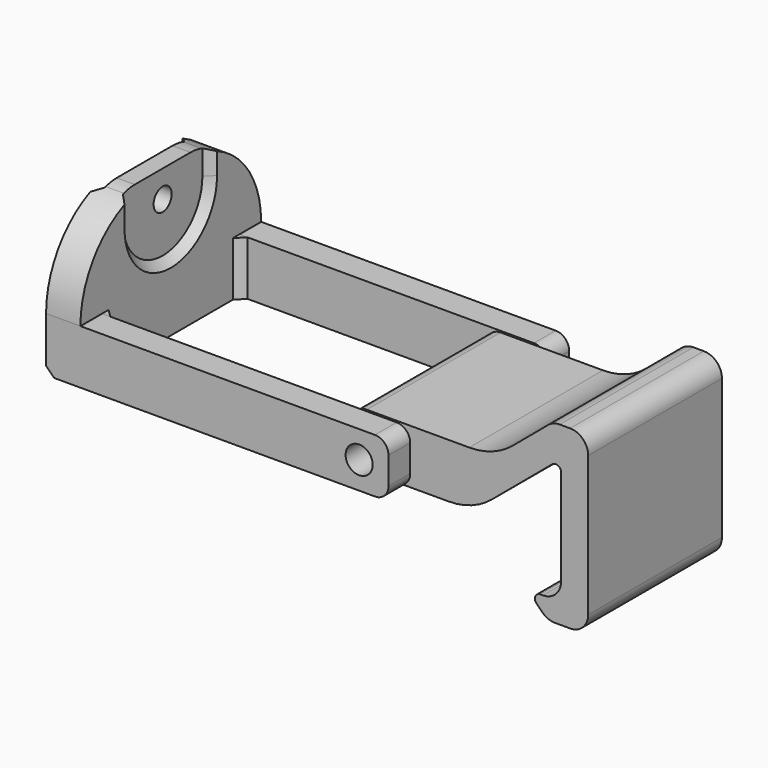
from build123d import *

# Parameters (mm, degrees)
F2_R          = 1.5
F5_DEPTH      = 12.5
F3_W          = 57.0000079349
F3_H          = 35
F3_W_2        = 5.9000002086
F3_H_2        = 3.0000003055
F6_DEPTH      = 25
F0_W          = 40
F0_H          = 30
F0_R          = 1.2500888111
F7_DEPTH      = 2
F8_DEPTH      = 1
F9_DEPTH      = 0.1
F10_DEPTH     = 0.1
F11_T4_DEPTH  = 8.3145145654
F11_T9_DEPTH  = 8.3145145654
F11_T11_DEPTH = 29.6290293933
F11_T16_ANGLE = 180
F11_T21_ANGLE = 180
F11_T26_DEPTH = 5.2499087538
F11_T31_DEPTH = 5.2499087441
F11_T36_DEPTH = 5.2499087441
F11_T41_DEPTH = 5.2499087538
F4_R          = 1.5
F12_DEPTH     = 9.25
F13_R         = 2
F14_R         = 7.5
F15_R         = 0.6
F1_W          = 40
F1_H          = 30
F16_DEPTH     = 12.5
F17_R         = 5


# Not quite as in the source:
# - a fillet or chamfer that OpenCascade refuses, or shapes differently, is made with other operations: its cross-section is extruded or revolved along the edge and cut away or added
# - ends of sketch curves that miss each other by under 0.0002 mm in the source are joined


with BuildPart() as f5:
    # F2 (on Front) → F5 (new body, symmetric)
    with BuildSketch(Plane.XZ):
        with BuildLine():
            Line((-6.5000004037, -1.225e-07), (34.4999995679, -1.225e-07))
            ThreePointArc((34.4999995679, -1.225e-07), (35.5606597229, 0.4393396988), (35.9999995441, 1.4999998538))
            Line((35.9999995441, 1.4999998538), (35.9999995441, 4.4999998063))
            ThreePointArc((35.9999995441, 4.4999998063), (35.5606597229, 5.5606599613), (34.4999995679, 5.9999997825))
            Line((34.4999995706, 5.9999997825), (1.9999998119, 5.9999998409))
            Line((1.9999998119, 5.999999905), (1.9999998119, 16))
            Line((1.9999998119, 16), (-2.000000095, 16))
            Line((-2.000000095, 16), (-2.000000095, 5.9999998557))
            Line((-2.000000095, 5.9999997745), (-6.500000401, 5.9999997825))
            ThreePointArc((-6.5000004037, 5.9999997825), (-7.5606605587, 5.5606599613), (-8.00000038, 4.4999998063))
            Line((-8.00000038, 4.4999998063), (-8.00000038, 1.4999998538))
            ThreePointArc((-8.00000038, 1.4999998538), (-7.5606605587, 0.4393396988), (-6.5000004037, -1.225e-07))
        make_face()
        with Locations((-4.7500003907, 2.9999998668)):
            Circle(F2_R, mode=Mode.SUBTRACT)
        with Locations((32.7499995548, 2.99999983)):
            Circle(F2_R, mode=Mode.SUBTRACT)
    extrude(amount=F5_DEPTH, both=True)

    # F3 (on Top) → F6 (cut)
    with BuildSketch(Plane.XY):
        with Locations((15.4999917634, -7.45e-08)):
            Rectangle(F3_W, F3_H)
        Polygon((-7.9000002086, 12.5), (-2, 12.5), (1.9999999069, 12.5), (35.9999998473, 12.5), (35.9999998473, 9.4999996945), (1.9999999069, 9.4999996945), (1.9999999069, -9.4999996945), (35.9999998473, -9.4999996945), (35.9999998473, -12.5), (1.9999999069, -12.5), (-2, -12.5), (-7.9000002086, -12.5), (-7.9000002086, -9.4999996945), (-2, -9.4999996945), (-2, 9.4999996945), (-7.9000002086, 9.4999996945), align=None, mode=Mode.SUBTRACT)
        with Locations((-4.9500001043, 10.9999998473)):
            Rectangle(F3_W_2, F3_H_2)
        with Locations((-4.9500001043, -10.9999998473)):
            Rectangle(F3_W_2, F3_H_2)
    extrude(amount=F6_DEPTH, mode=Mode.SUBTRACT)

    # F0 (on Right) → F7 (cut, symmetric)
    with BuildSketch(Plane.YZ):
        with Locations((4.47e-07, 7.9853728972)):
            Rectangle(F0_W, F0_H)
        with BuildLine():
            Line((12.5, -0.0146211902), (-12.5, -0.0146211902))
            Line((-12.5, -0.0146211902), (-12.5, 7.9853788098))
            ThreePointArc((-12.5, 7.9853788098), (-10.5000000081, 13.276881496), (-5.5, 15.9226329138))
            ThreePointArc((-5.5, 15.9226329138), (-5.000983204, 15.9696770716), (-4.4999998063, 15.9853790035))
            Line((-4.4999998063, 15.9853790035), (4.4999998063, 15.9853790035))
            ThreePointArc((4.4999998063, 15.9853790035), (5.000983204, 15.9696770716), (5.5, 15.9226329138))
            ThreePointArc((5.5, 15.9226329138), (10.5000000081, 13.276881496), (12.5, 7.9853788098))
            Line((12.5, 7.9853788098), (12.5, -0.0146211902))
        make_face(mode=Mode.SUBTRACT)
        with BuildLine():
            ThreePointArc((-4.4999998063, 15.9853790035), (-5.000983204, 15.9696770716), (-5.5, 15.9226329138))
            Line((-5.5, 15.9226329138), (-5.5, 12.9872388524))
            ThreePointArc((-5.5, 12.9872388524), (0, 7.4872388524), (5.5, 12.9872388524))
            Line((5.5, 12.9872388524), (5.5, 15.9226329138))
            ThreePointArc((5.5, 15.9226329138), (5.000983204, 15.9696770716), (4.4999998063, 15.9853790035))
            Line((4.4999998063, 15.9853790035), (-4.4999998063, 15.9853790035))
        make_face()
        with Locations((0, 12.9872388524)):
            Circle(F0_R, mode=Mode.SUBTRACT)
        with Locations((0, 12.9872388524)):
            Circle(F0_R)
    extrude(amount=F7_DEPTH, both=True, mode=Mode.SUBTRACT)

    # F0 (on Right) → F8 (join, symmetric)
    with BuildSketch(Plane.YZ):
        with BuildLine():
            ThreePointArc((-4.4999998063, 15.9853790035), (-5.000983204, 15.9696770716), (-5.5, 15.9226329138))
            Line((-5.5, 15.9226329138), (-5.5, 12.9872388524))
            ThreePointArc((-5.5, 12.9872388524), (0, 7.4872388524), (5.5, 12.9872388524))
            Line((5.5, 12.9872388524), (5.5, 15.9226329138))
            ThreePointArc((5.5, 15.9226329138), (5.000983204, 15.9696770716), (4.4999998063, 15.9853790035))
            Line((4.4999998063, 15.9853790035), (-4.4999998063, 15.9853790035))
        make_face()
        with Locations((0, 12.9872388524)):
            Circle(F0_R, mode=Mode.SUBTRACT)
    extrude(amount=F8_DEPTH, both=True)

    # F9 (cut): a face of the model
    f9_faces = [f5.faces().sort_by_distance(p)[0] for p in [
        (1.9999998119, 0, 6.6984167583),
    ]]
    extrude(f9_faces, amount=-F9_DEPTH, mode=Mode.SUBTRACT)

    # F10 (cut): a face of the model
    f10_faces = [f5.faces().sort_by_distance(p)[0] for p in [
        (-2.000000095, 0, 6.2419959068),
    ]]
    extrude(f10_faces, amount=-F10_DEPTH, mode=Mode.SUBTRACT)

    # F11: chamfer of 0.9 on 9 edges, made by hand


with BuildPart() as f11_tool2:
    # F11_s3 → F11_t4 (new body)
    with BuildSketch(Plane.XY.offset(-2.3145146924)):
        with BuildLine():
            Line((1.8745439664, 8.5745438517), (2.8254557523, 9.5254555373))
            Line((2.8254557523, 9.5254555373), (2.8254557523, 9.5434555373))
            ThreePointArc((2.8254557523, 9.5434555373), (2.3627278296, 9.5179996945), (1.8999999069, 9.5179996945))
            Line((1.8999999069, 9.5179996945), (1.8819999069, 9.4999996945))
            ThreePointArc((1.8819999069, 9.4999996945), (1.8819998119, 9.0372717731), (1.8565439664, 8.5745438517))
            Line((1.8565439664, 8.5745438517), (1.8745439664, 8.5745438517))
        make_face()
    extrude(amount=F11_T4_DEPTH)

    split(bisect_by=Plane.XY.offset(-1.225e-07), keep=Keep.TOP)


with BuildPart() as f5_1:
    add(f5.part)

    # F11_t1: union F11_tool2
    add(f11_tool2.part)


with BuildPart() as f11_tool7:
    # F11_s8 → F11_t9 (new body)
    with BuildSketch(Plane.XY.offset(-2.3145146924)):
        with BuildLine():
            Line((1.8745439664, -8.5745438517), (2.8254557523, -9.5254555373))
            Line((2.8254557523, -9.5254555373), (2.8254557523, -9.5434555373))
            ThreePointArc((2.8254557523, -9.5434555373), (2.3627278296, -9.5179996945), (1.8999999069, -9.5179996945))
            Line((1.8999999069, -9.5179996945), (1.8819999069, -9.4999996945))
            ThreePointArc((1.8819999069, -9.4999996945), (1.8819998119, -9.0372717731), (1.8565439664, -8.5745438517))
            Line((1.8565439664, -8.5745438517), (1.8745439664, -8.5745438517))
        make_face()
    extrude(amount=F11_T9_DEPTH)

    split(bisect_by=Plane.XY.offset(-1.225e-07), keep=Keep.TOP)


with BuildPart() as f5_2:
    add(f5_1.part)

    # F11_t6: union F11_tool7
    add(f11_tool7.part)

    # F11_s12 → F11_t11 (cut)
    with BuildSketch(Plane.XZ.offset(-14.8145146966)):
        with BuildLine():
            Line((-1.9254559387, 0.9254558445), (-0.9745441563, -0.025455967))
            Line((-0.9745441563, -0.025455967), (-0.9745441563, -0.043455967))
            ThreePointArc((-0.9745441563, -0.043455967), (-1.4372720781, -0.0180001225), (-1.9, -0.018))
            Line((-1.9, -0.018), (-1.918, 0))
            ThreePointArc((-1.918, 0), (-1.918000095, 0.4627279223), (-1.9434559387, 0.9254558445))
            Line((-1.9434559387, 0.9254558445), (-1.9254559387, 0.9254558445))
        make_face()
    extrude(amount=F11_T11_DEPTH, mode=Mode.SUBTRACT)


with BuildPart() as f11_tool14:
    # F11_s15 → F11_t16 (revolve)
    with BuildSketch(Plane.XY.offset(12.9872388524)):
        with BuildLine():
            Line((0.9745441585, -5.4745441532), (1.9254556533, -6.4254558468))
            Line((1.9254556533, -6.4254558468), (1.9434556533, -6.4254558468))
            ThreePointArc((1.9434556533, -6.4254558468), (1.9179998119, -5.9627279234), (1.918, -5.5))
            Line((1.918, -5.5), (1.9, -5.482))
            ThreePointArc((1.9, -5.482), (1.4372720793, -5.482), (0.9745441585, -5.4565441532))
            Line((0.9745441585, -5.4565441532), (0.9745441585, -5.4745441532))
        make_face()
    revolve(axis=Axis((1.9, 0, 12.9872388524), (1, 0, 0)), revolution_arc=F11_T16_ANGLE)

    split(bisect_by=Plane.YZ.offset(1), keep=Keep.TOP)


with BuildPart() as f5_3:
    add(f5_2.part)

    # F11_t13: cut F11_tool14
    add(f11_tool14.part, mode=Mode.SUBTRACT)


with BuildPart() as f11_tool19:
    # F11_s20 → F11_t21 (revolve)
    with BuildSketch(Plane.XY.offset(12.9872388524)):
        with BuildLine():
            Line((-1.9254559405, -6.4254558428), (-0.9745441545, -5.4745441572))
            Line((-0.9745441545, -5.4745441572), (-0.9745441545, -5.4565441572))
            ThreePointArc((-0.9745441545, -5.4565441572), (-1.4372720773, -5.482), (-1.9, -5.482))
            Line((-1.9, -5.482), (-1.918, -5.5))
            ThreePointArc((-1.918, -5.5), (-1.918000095, -5.9627279214), (-1.9434559405, -6.4254558428))
            Line((-1.9434559405, -6.4254558428), (-1.9254559405, -6.4254558428))
        make_face()
    revolve(axis=Axis((-1.9, 0, 12.9872388524), (1, 0, 0)), revolution_arc=F11_T21_ANGLE)

    split(bisect_by=Plane.YZ.offset(-1), keep=Keep.BOTTOM)


with BuildPart() as f5_4:
    add(f5_3.part)

    # F11_t18: cut F11_tool19
    add(f11_tool19.part, mode=Mode.SUBTRACT)


with BuildPart() as f11_tool24:
    # F11_s25 → F11_t26 (new body)
    with BuildSketch(Plane.XY.offset(12.9872388524)):
        with BuildLine():
            Line((-1.9254559405, 6.4254558428), (-0.9745441545, 5.4745441572))
            Line((-0.9745441545, 5.4745441572), (-0.9745441545, 5.4565441572))
            ThreePointArc((-0.9745441545, 5.4565441572), (-1.4372720773, 5.482), (-1.9, 5.482))
            Line((-1.9, 5.482), (-1.918, 5.5))
            ThreePointArc((-1.918, 5.5), (-1.918000095, 5.9627279214), (-1.9434559405, 6.4254558428))
            Line((-1.9434559405, 6.4254558428), (-1.9254559405, 6.4254558428))
        make_face()
    extrude(amount=F11_T26_DEPTH)

    split(bisect_by=Plane.YZ.offset(-1), keep=Keep.BOTTOM)


with BuildPart() as f5_5:
    add(f5_4.part)

    # F11_t23: cut F11_tool24
    add(f11_tool24.part, mode=Mode.SUBTRACT)


with BuildPart() as f11_tool29:
    # F11_s30 → F11_t31 (new body)
    with BuildSketch(Plane.XY.offset(12.9872388524)):
        with BuildLine():
            Line((1.9254556533, 6.4254558468), (0.9745441585, 5.4745441532))
            Line((0.9745441585, 5.4745441532), (0.9745441585, 5.4565441532))
            ThreePointArc((0.9745441585, 5.4565441532), (1.4372720793, 5.482), (1.9, 5.482))
            Line((1.9, 5.482), (1.918, 5.5))
            ThreePointArc((1.918, 5.5), (1.9179998119, 5.9627279234), (1.9434556533, 6.4254558468))
            Line((1.9434556533, 6.4254558468), (1.9254556533, 6.4254558468))
        make_face()
    extrude(amount=F11_T31_DEPTH)

    split(bisect_by=Plane.YZ.offset(1), keep=Keep.TOP)


with BuildPart() as f5_6:
    add(f5_5.part)

    # F11_t28: cut F11_tool29
    add(f11_tool29.part, mode=Mode.SUBTRACT)


with BuildPart() as f11_tool34:
    # F11_s35 → F11_t36 (new body)
    with BuildSketch(Plane.XY.offset(18.2371475965)):
        with BuildLine():
            Line((0.9745441585, -5.4745441532), (1.9254556533, -6.4254558468))
            Line((1.9254556533, -6.4254558468), (1.9434556533, -6.4254558468))
            ThreePointArc((1.9434556533, -6.4254558468), (1.9179998119, -5.9627279234), (1.918, -5.5))
            Line((1.918, -5.5), (1.9, -5.482))
            ThreePointArc((1.9, -5.482), (1.4372720793, -5.482), (0.9745441585, -5.4565441532))
            Line((0.9745441585, -5.4565441532), (0.9745441585, -5.4745441532))
        make_face()
    extrude(amount=-F11_T36_DEPTH)

    split(bisect_by=Plane.YZ.offset(1), keep=Keep.TOP)


with BuildPart() as f5_7:
    add(f5_6.part)

    # F11_t33: cut F11_tool34
    add(f11_tool34.part, mode=Mode.SUBTRACT)


with BuildPart() as f11_tool39:
    # F11_s40 → F11_t41 (new body)
    with BuildSketch(Plane.XY.offset(18.2371476062)):
        with BuildLine():
            Line((-1.9254559405, -6.4254558428), (-0.9745441545, -5.4745441572))
            Line((-0.9745441545, -5.4745441572), (-0.9745441545, -5.4565441572))
            ThreePointArc((-0.9745441545, -5.4565441572), (-1.4372720773, -5.482), (-1.9, -5.482))
            Line((-1.9, -5.482), (-1.918, -5.5))
            ThreePointArc((-1.918, -5.5), (-1.918000095, -5.9627279214), (-1.9434559405, -6.4254558428))
            Line((-1.9434559405, -6.4254558428), (-1.9254559405, -6.4254558428))
        make_face()
    extrude(amount=-F11_T41_DEPTH)

    split(bisect_by=Plane.YZ.offset(-1), keep=Keep.BOTTOM)


with BuildPart() as f5_8:
    add(f5_7.part)

    # F11_t38: cut F11_tool39
    add(f11_tool39.part, mode=Mode.SUBTRACT)

    # F1 (on Right) → F16 (cut, symmetric)
    with BuildSketch(Plane.YZ):
        with Locations((4.47e-07, 7.9853728972)):
            Rectangle(F1_W, F1_H)
        with BuildLine():
            Line((-4.4999998063, 15.9853790035), (4.4999998063, 15.9853790035))
            ThreePointArc((4.4999998063, 15.9853790035), (10.2533424116, 12.3974172553), (12.5, 5.9999997825))
            Line((12.5, 5.9999997825), (12.5, -0.0146211902))
            Line((12.5, -0.0146211902), (-12.5, -0.0146211902))
            Line((-12.5, -0.0146211902), (-12.5, 5.9999997825))
            ThreePointArc((-12.5, 5.9999997825), (-10.2533424116, 12.3974172553), (-4.4999998063, 15.9853790035))
        make_face(mode=Mode.SUBTRACT)
    extrude(amount=F16_DEPTH, both=True, mode=Mode.SUBTRACT)

    # F17
    f17_edges = [f5_8.edges().sort_by_distance(p)[0] for p in [
        (0, -4.5, 15.985379),
        (0, 4.5, 15.985379),
    ]]
    fillet(f17_edges, radius=F17_R)


with BuildPart() as f12:
    # F4 (on Front) → F12 (new body, symmetric)
    with BuildSketch(Plane.XZ):
        with BuildLine():
            ThreePointArc((29.4999995655, 1.4999998538), (29.9393393859, 0.4393396997), (30.9999995391, -1.225e-07))
            Line((30.9999995391, -1.225e-07), (42.7499995548, -1.436e-07))
            Line((42.7499995548, -1.436e-07), (52.5000281632, 8.1812452657))
            Line((52.5000281632, 8.1812452657), (52.5000281632, -5.7499710164))
            Line((52.5000281632, -5.7499710164), (48.7499994809, -5.7499708617))
            Line((48.7499994809, -5.7499708617), (51.0000307917, -8.0000022426))
            Line((51.0000307917, -8.0000022426), (55.5000305176, -8.0000024282))
            Line((55.5000305176, -8.0000024282), (55.5000305176, 11.5000018742))
            Line((55.5000305176, 11.5000018742), (51.6208254365, 11.5000018812))
            Line((51.6208254365, 11.5000018812), (45.0661781761, 5.9999997825))
            Line((45.0661781761, 5.9999997825), (30.9999995418, 5.9999997825))
            ThreePointArc((30.9999995418, 5.9999997825), (29.9393393868, 5.5606599613), (29.4999995655, 4.4999998063))
            Line((29.4999995655, 4.4999998063), (29.4999995655, 1.4999998538))
        make_face()
        with Locations((32.7499995548, 2.99999983)):
            Circle(F4_R, mode=Mode.SUBTRACT)
    extrude(amount=F12_DEPTH, both=True)

    # F13
    f13_edges = [f12.edges().sort_by_distance(p)[0] for p in [
        (51.620825, 0, 11.500002),
        (55.500031, 0, 11.500002),
        (55.500031, 0, -8.000002),
        (51.000031, 0, -8.000002),
        (52.500028, 0, -5.749971),
    ]]
    fillet(f13_edges, radius=F13_R)

    # F14
    f14_edges = [f12.edges().sort_by_distance(p)[0] for p in [
        (45.066178, 0, 6),
        (42.75, 0, 0),
    ]]
    fillet(f14_edges, radius=F14_R)

    # F15
    f15_edges = [f12.edges().sort_by_distance(p)[0] for p in [
        (52.500028, 0, 8.181245),
        (48.749999, 0, -5.749971),
    ]]
    fillet(f15_edges, radius=F15_R)


solid = Compound([f5_8.part, f12.part])
